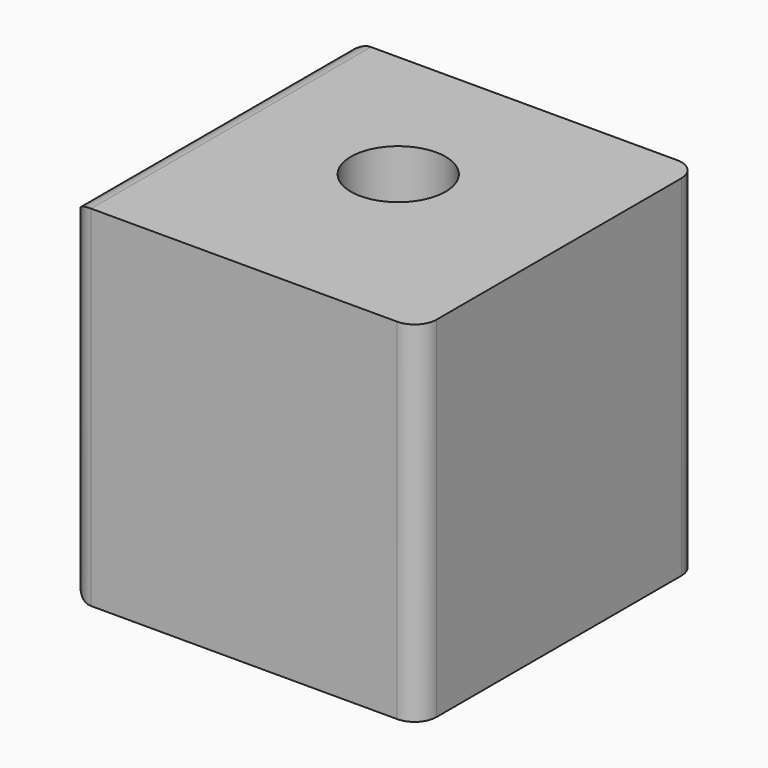
from build123d import *

# Parameters (mm, degrees)
F0_W     = 80
F0_H     = 80
F1_DEPTH = 80
F3_R     = 5
F2_R     = 10.8374332622
F4_DEPTH = 80.001


with BuildPart() as f1:
    # F0 (on Top) → F1 (new body)
    with BuildSketch(Plane.XY):
        with Locations((-41.452800855, 28.8035999984)):
            Rectangle(F0_W, F0_H)
    extrude(amount=F1_DEPTH)

    # F3
    f3_edges = [f1.edges().sort_by_distance(p)[0] for p in [
        (-81.452801, -11.1964, 40),
        (-1.452801, -11.1964, 40),
        (-1.452801, 68.8036, 40),
        (-81.452801, 68.8036, 40),
        (-81.452801, 28.8036, 0),
        (-81.452801, 28.8036, 80),
    ]]
    fillet(f3_edges, radius=F3_R)

    # F2 (on face) → F4 (cut, through all)
    with BuildSketch(Plane.XY.offset(80)):
        with Locations((-41.9264025986, 33.4499999881)):
            Circle(F2_R)
    extrude(amount=-F4_DEPTH, mode=Mode.SUBTRACT)


solid = f1.part
